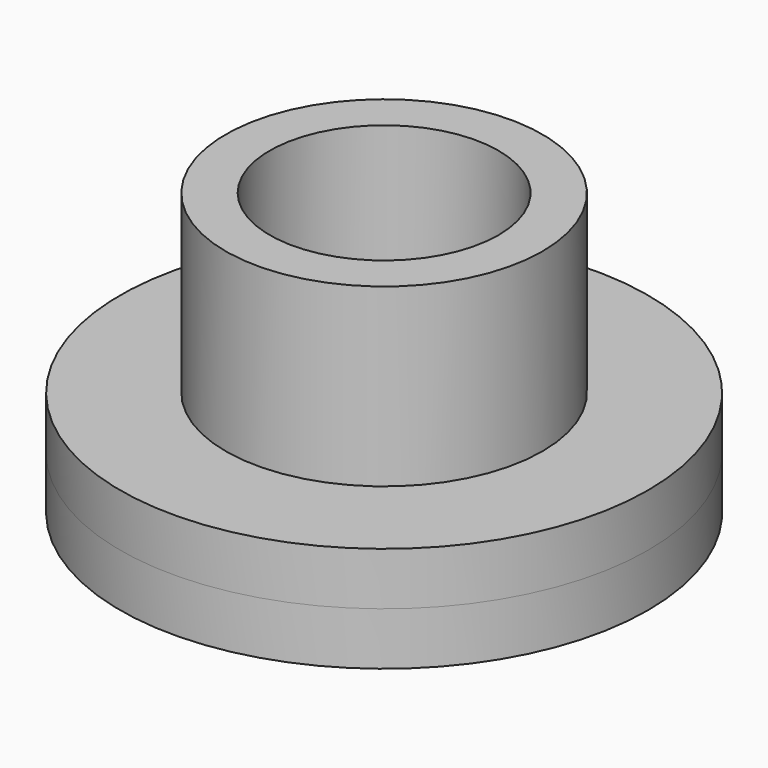
from build123d import *

# Parameters (mm, degrees)
F0_R     = 15
F0_R_2   = 11.5
F1_DEPTH = 3
F0_R_3   = 9
F0_R_4   = 6.5
F2_R     = 15
F2_R_2   = 11.5
F2_R_3   = 6.5
F3_DEPTH = 3
F4_R     = 9
F4_R_2   = 6.5
F5_DEPTH = 10


# Not quite as in the source:
# - a feature names something its author has since deleted; it is built from what else it names


with BuildPart() as f1:
    # F0 (on Top) → F1 (new body)
    with BuildSketch(Plane.XY):
        Circle(F0_R)
        Circle(F0_R_2, mode=Mode.SUBTRACT)
    extrude(amount=F1_DEPTH)


with BuildPart() as f1b:
    # F0 (on Top) → F1, piece 2 (new body)
    with BuildSketch(Plane.XY):
        Circle(F0_R_3)
        Circle(F0_R_4, mode=Mode.SUBTRACT)
    extrude(amount=F1_DEPTH)


with BuildPart() as f3:
    # F2 (on face) → F3 (new body)
    with BuildSketch(Plane.XY.offset(3)):
        Circle(F2_R)
        Circle(F2_R_2, mode=Mode.SUBTRACT)
        Circle(F2_R_2)
        Circle(F2_R_3, mode=Mode.SUBTRACT)
    extrude(amount=F3_DEPTH)

    # F4 (on face) → F5 (join)
    with BuildSketch(Plane.XY.offset(6)):
        Circle(F4_R)
        Circle(F4_R_2, mode=Mode.SUBTRACT)
    extrude(amount=F5_DEPTH)


solid = Compound([f1.part, f1b.part, f3.part])
